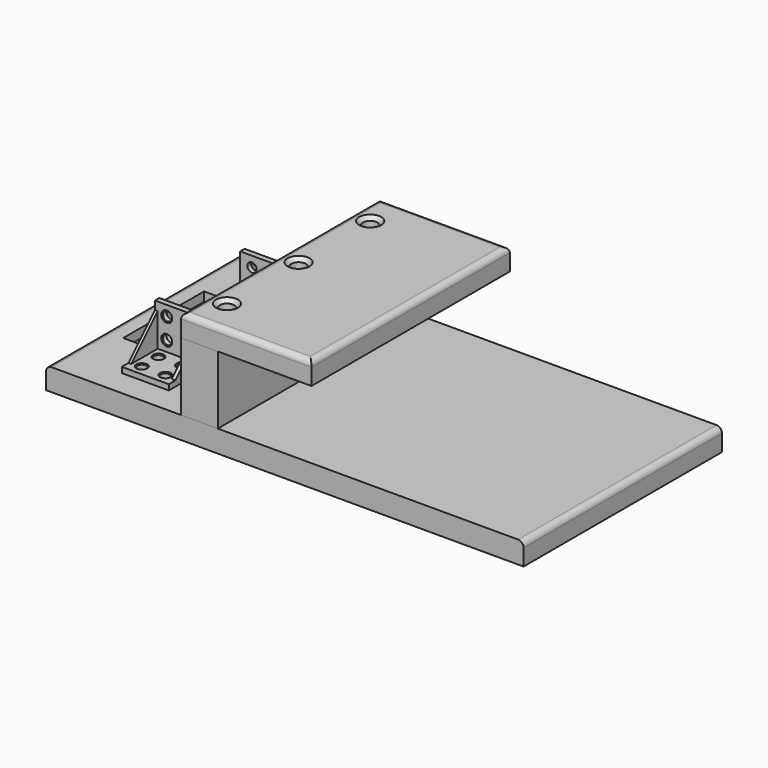
from build123d import *

# Parameters (mm, degrees)
F1_DEPTH        = 6
F2_W            = 63.5
F2_H            = 55
F3_DEPTH        = 5
F4_W            = 20
F4_H            = 135
F5_DEPTH        = 37
F7_D            = 8
F7_DEPTH        = 12
F7_CSINK_D      = 12
F7_CSINK_ANGLE  = 90
F7_TIP          = 2.4034424761
F8_W            = 71
F8_H            = 135
F9_DEPTH        = 12
F11_D           = 8
F11_DEPTH       = 12
F11_CSINK_D     = 12
F11_CSINK_ANGLE = 90
F11_TIP         = 2.4034424761
F12_R           = 3
F12_2_R         = 3
F13_W           = 25.6
F13_H           = 25.6
F14_DEPTH       = 3
F15_W           = 25.6
F15_H           = 3
F16_DEPTH       = 22.6
F18_D           = 5
F18_DEPTH       = 3
F18_CSINK_D     = 6
F18_CSINK_ANGLE = 90
F18_TIP         = 1.5021515476
F20_D           = 5
F20_DEPTH       = 3
F20_CSINK_D     = 6
F20_CSINK_ANGLE = 90
F20_TIP         = 1.5021515476
F22_DEPTH       = 1.5
F24_DEPTH       = 2


# Not quite as in the source:
# - a feature names something its author has since deleted; it is built from what else it names


with BuildPart() as f1:
    # F0 (on Top) → F1 (new body, symmetric)
    with BuildSketch(Plane.XY):
        Polygon((125, -67.5), (125, 67.5), (-125, 67.5), (-135, 67.5), (-135, -67.5), align=None)
    extrude(amount=F1_DEPTH, both=True)

    # F2 (on face) → F3 (cut)
    with BuildSketch(Plane.XY.offset(6)):
        with Locations((-93.25, 0)):
            Rectangle(F2_W, F2_H)
    extrude(amount=-F3_DEPTH, mode=Mode.SUBTRACT)

    # F7
    with Locations(Plane(origin=(0, 0, -6), x_dir=(1, 0, 0), z_dir=(0, 0, -1))):
        with Locations((-51.5, 33.75), (-51.5, 0), (-51.5, -33.75)):
            CounterSinkHole(F7_D / 2, F7_CSINK_D / 2, depth=F7_DEPTH, counter_sink_angle=F7_CSINK_ANGLE)
            with Locations((0, 0, -(F7_DEPTH + F7_TIP / 2))):  # 118° drill point
                Cone(0, F7_D / 2, F7_TIP, mode=Mode.SUBTRACT)

    # F12
    f12_edges = [f1.edges().sort_by_distance(p)[0] for p in [
        (125, 0, 6),
        (-135, 0, 6),
    ]]
    fillet(f12_edges, radius=F12_R)


with BuildPart() as f5:
    # F4 (on face) → F5 (new body)
    with BuildSketch(Plane.XY.offset(6)):
        with Locations((-51.5, 0)):
            Rectangle(F4_W, F4_H)
    extrude(amount=F5_DEPTH)


with BuildPart() as f9:
    # F8 (on face) → F9 (new body)
    with BuildSketch(Plane.XY.offset(43)):
        with Locations((-26, 0)):
            Rectangle(F8_W, F8_H)
    extrude(amount=F9_DEPTH)

    # F11
    with Locations(Plane.XY.offset(55)):
        with Locations((-51.5, 48.75), (-51.5, 0), (-51.5, -48.75)):
            CounterSinkHole(F11_D / 2, F11_CSINK_D / 2, depth=F11_DEPTH, counter_sink_angle=F11_CSINK_ANGLE)
            with Locations((0, 0, -(F11_DEPTH + F11_TIP / 2))):  # 118° drill point
                Cone(0, F11_D / 2, F11_TIP, mode=Mode.SUBTRACT)

    # F12#2
    f12_2_edges = [f9.edges().sort_by_distance(p)[0] for p in [
        (9.5, 0, 55),
        (-26, -67.5, 55),
        (-26, 67.5, 55),
        (-61.5, 0, 55),
    ]]
    fillet(f12_2_edges, radius=F12_2_R)


with BuildPart() as f14:
    # F13 (on face) → F14 (new body)
    with BuildSketch(Plane.XY.offset(6)):
        with Locations((-92.5, 40.3)):
            Rectangle(F13_W, F13_H)
    extrude(amount=F14_DEPTH)

    # F15 (on face) → F16 (join)
    with BuildSketch(Plane.XY.offset(9)):
        with Locations((-92.5, 29)):
            Rectangle(F15_W, F15_H)
    extrude(amount=F16_DEPTH)

    # F18
    with Locations(Plane(origin=(0, 30.5, 0), x_dir=(-1, 0, 0), z_dir=(0, 1, 0))):
        with Locations((86.1, 25.95), (98.9, 25.95), (86.1, 14.65), (98.9, 14.65)):
            CounterSinkHole(F18_D / 2, F18_CSINK_D / 2, depth=F18_DEPTH, counter_sink_angle=F18_CSINK_ANGLE)
            with Locations((0, 0, -(F18_DEPTH + F18_TIP / 2))):  # 118° drill point
                Cone(0, F18_D / 2, F18_TIP, mode=Mode.SUBTRACT)

    # F20
    with Locations(Plane.XY.offset(9)):
        with Locations((-86.1, 36.15), (-98.9, 36.15), (-98.9, 47.45), (-86.1, 47.45)):
            CounterSinkHole(F20_D / 2, F20_CSINK_D / 2, depth=F20_DEPTH, counter_sink_angle=F20_CSINK_ANGLE)
            with Locations((0, 0, -(F20_DEPTH + F20_TIP / 2))):  # 118° drill point
                Cone(0, F20_D / 2, F20_TIP, mode=Mode.SUBTRACT)

    # F21 (on face) → F22 (join)
    with BuildSketch(Plane(origin=(-105.3, 0, 0), x_dir=(0, -1, 0), z_dir=(-1, 0, 0))):
        Polygon((-30.5, 9), (-30.5, 27.1), (-48.6, 9), align=None)
    extrude(amount=-F22_DEPTH)

    # F23 (on face) → F24 (join)
    with BuildSketch(Plane.YZ.offset(-79.7)):
        Polygon((30.5, 27.1), (30.5, 9), (48.6, 9), align=None)
    extrude(amount=-F24_DEPTH)


with BuildPart() as f25_1:
    # F25: instance of F14
    add(f14.part.mirror(Plane.XZ))


solid = Compound([f1.part, f5.part, f9.part, f14.part, f25_1.part])
